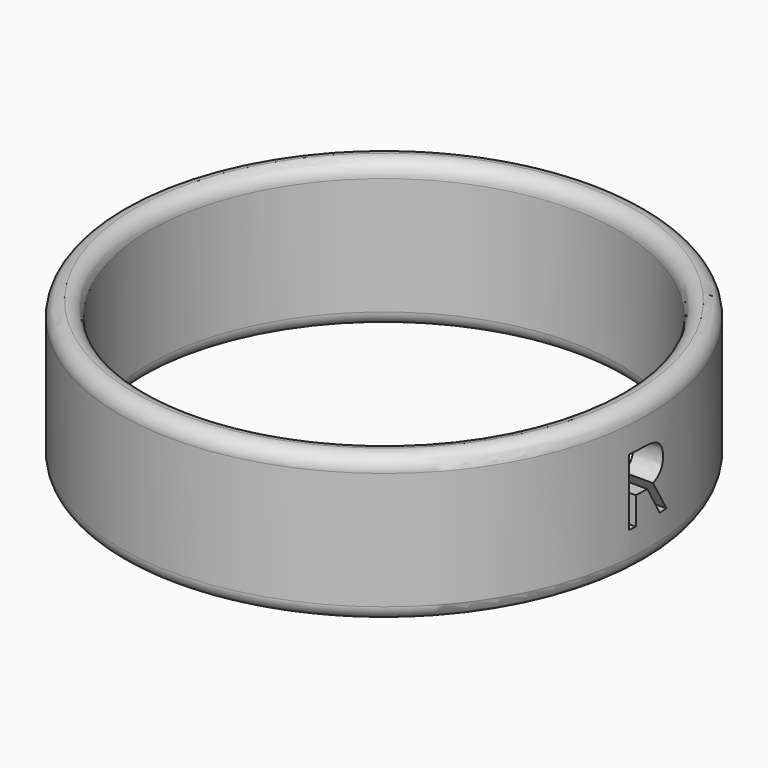
from build123d import *

# Parameters (mm, degrees)
F0_R     = 9
F0_R_2   = 8
F1_DEPTH = 5
F2_R     = 0.49999
F3_R     = 0.49999
F6_DEPTH = 25


# Not quite as in the source:
# - a fillet or chamfer is up to 0.001 mm smaller than in the source, because OpenCascade refuses the exact size


with BuildPart() as f1:
    # F0 (on Top) → F1 (new body)
    with BuildSketch(Plane.XY):
        Circle(F0_R)
        Circle(F0_R_2, mode=Mode.SUBTRACT)
    extrude(amount=F1_DEPTH)

    # F2 (radius 0.5 in the source; OpenCascade refuses exactly that, so slightly less here)
    f2_edges = [f1.edges().sort_by_distance(p)[0] for p in [
        (-8, 0, 5),
        (-9, 0, 5),
    ]]
    fillet(f2_edges, radius=F2_R)

    # F3 (radius 0.5 in the source; OpenCascade refuses exactly that, so slightly less here)
    f3_edges = [f1.edges().sort_by_distance(p)[0] for p in [
        (-8, 0, 0),
        (-9, 0, 0),
    ]]
    fillet(f3_edges, radius=F3_R)

    # F5 (on offset) → F6 (cut)
    with BuildSketch(Plane.YZ.offset(25)):
        with BuildLine():
            Line((-0.5083193487, 1.3498821063), (-0.5083193487, 2.2919357963))
            Line((-0.5083193487, 2.2919357963), (-0.0353092327, 2.2919357963))
            Line((-0.0353092327, 2.2919357963), (0.5130651784, 1.3498821063))
            Line((0.5130651784, 1.3498821063), (0.8244387138, 1.3498821063))
            Line((0.8244387138, 1.3498821063), (0.2091289089, 2.3677959092))
            add(Edge.make_bspline(
                [(0.6647854042, 2.9751726304), (0.6647854042, 2.5259617656), (0.2091289089, 2.3677959092)],
                knots=[0, 0, 0, 1, 1, 1], degree=2))
            add(Edge.make_bspline(
                [(0.465714585, 3.4556200122), (0.6647854042, 3.2959667027), (0.6647854042, 2.9751726304)],
                knots=[0, 0, 0, 1, 1, 1], degree=2))
            add(Edge.make_bspline(
                [(-0.1503389465, 3.6152733218), (0.2666437658, 3.6152733218), (0.465714585, 3.4556200122)],
                knots=[0, 0, 0, 1, 1, 1], degree=2))
            Line((-0.1503389465, 3.6152733218), (-0.7715985641, 3.6152733218))
            Line((-0.7715985641, 3.6152733218), (-0.7715985641, 1.3498821063))
            Line((-0.7715985641, 1.3498821063), (-0.5083193487, 1.3498821063))
        make_face()
        Polygon((-0.5905224825, 2.4278266355), (-0.5905224825, 3.4481487237), (0, 3.4917523153), (0.4821238399, 3.2650141511), (0.4821238399, 2.7940962464), (0.1768992952, 2.4278266355), align=None, mode=Mode.SUBTRACT)
        Polygon((0, 3.4917523153), (-0.5905224825, 3.4481487237), (-0.5905224825, 2.4278266355), (0.1768992952, 2.4278266355), (0.4821238399, 2.7940962464), (0.4821238399, 3.2650141511), align=None)
        with BuildLine():
            Line((-0.1468682223, 2.5180286819), (-0.5083193487, 2.5180286819))
            Line((-0.5083193487, 2.5180286819), (-0.5083193487, 3.3842222589))
            Line((-0.5083193487, 3.3842222589), (-0.1657092961, 3.3842222589))
            add(Edge.make_bspline(
                [(0.2597023175, 3.2850587126), (0.1273189832, 3.3842222589), (-0.1657092961, 3.3842222589)],
                knots=[0, 0, 0, 1, 1, 1], degree=2))
            add(Edge.make_bspline(
                [(0.3920856519, 2.9612897339), (0.3920856519, 3.1858951663), (0.2597023175, 3.2850587126)],
                knots=[0, 0, 0, 1, 1, 1], degree=2))
            add(Edge.make_bspline(
                [(0.2619334973, 2.6288439449), (0.3920856519, 2.7396592079), (0.3920856519, 2.9612897339)],
                knots=[0, 0, 0, 1, 1, 1], degree=2))
            add(Edge.make_bspline(
                [(-0.1468682223, 2.5180286819), (0.1317813428, 2.5180286819), (0.2619334973, 2.6288439449)],
                knots=[0, 0, 0, 1, 1, 1], degree=2))
        make_face(mode=Mode.SUBTRACT)
        with BuildLine():
            Line((-0.5083193487, 3.3842222589), (-0.5083193487, 2.5180286819))
            Line((-0.5083193487, 2.5180286819), (-0.1468682223, 2.5180286819))
            add(Edge.make_bspline(
                [(-0.1468682223, 2.5180286819), (0.1317813428, 2.5180286819), (0.2619334973, 2.6288439449)],
                knots=[0, 0, 0, 1, 1, 1], degree=2))
            add(Edge.make_bspline(
                [(0.2619334973, 2.6288439449), (0.3920856519, 2.7396592079), (0.3920856519, 2.9612897339)],
                knots=[0, 0, 0, 1, 1, 1], degree=2))
            add(Edge.make_bspline(
                [(0.3920856519, 2.9612897339), (0.3920856519, 3.1858951663), (0.2597023175, 3.2850587126)],
                knots=[0, 0, 0, 1, 1, 1], degree=2))
            add(Edge.make_bspline(
                [(0.2597023175, 3.2850587126), (0.1273189832, 3.3842222589), (-0.1657092961, 3.3842222589)],
                knots=[0, 0, 0, 1, 1, 1], degree=2))
            Line((-0.1657092961, 3.3842222589), (-0.5083193487, 3.3842222589))
        make_face()
    extrude(amount=-F6_DEPTH, mode=Mode.SUBTRACT)


solid = f1.part
